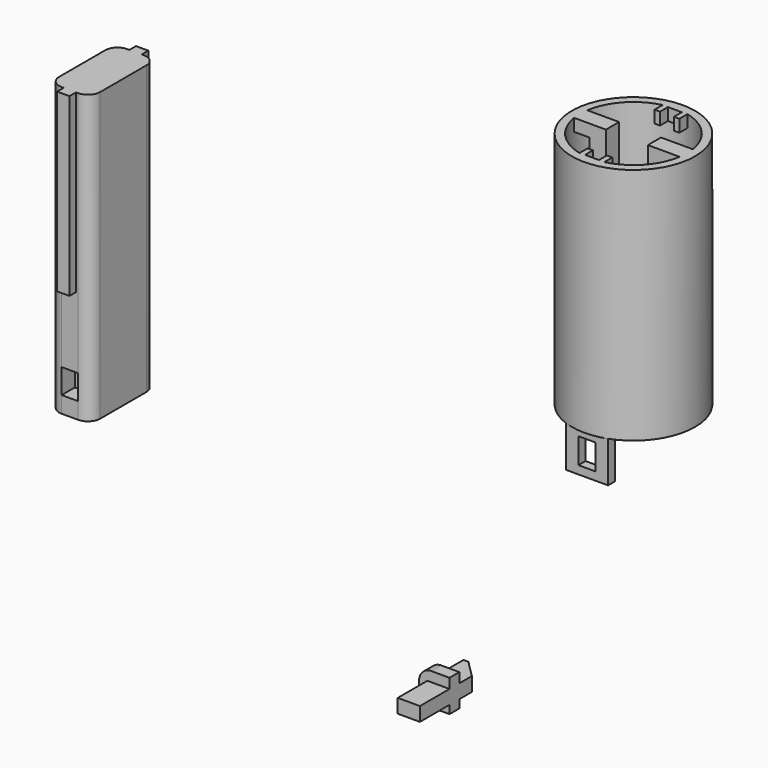
from build123d import *

# Parameters (mm, degrees)
F0_R           = 7.5
F1_DEPTH       = 29
F2_R           = 6.5
F3_DEPTH       = 30
F4_R           = 7.5
F4_R_2         = 6.5
F5_DEPTH       = 2
F7_DEPTH       = 35
F9_DEPTH       = 1.5
F10_W          = 1.5
F10_H          = 1
F11_DEPTH      = 13.6
F13_DEPTH      = 25
F14_R          = 1.5
F15_W          = 1
F15_H          = 3
F16_DEPTH      = 2
F17_W          = 5.1
F17_H          = 1.0742694599
F18_DEPTH      = 5
F19_W          = 2.1
F19_H          = 3.1
F20_DEPTH      = 25
F21_W          = 2.7
F21_H          = 1.7
F22_DEPTH      = 10
F24_DEPTH      = 25
F25_W          = 2
F25_H          = 2
F26_DEPTH      = 25.5
F27_W          = 3.7
F27_H          = 1.5
F28_DEPTH      = 1
F28_DEPTH_BACK = 2.9
F29_R          = 1.5


# Not quite as in the source:
# - a feature names something its author has since deleted; it is built from what else it names


with BuildPart() as f1:
    # F0 (on Top) → F1 (new body)
    with BuildSketch(Plane.XY):
        Circle(F0_R)
    extrude(amount=F1_DEPTH)

    # F2 (on Top) → F3 (cut)
    with BuildSketch(Plane.XY):
        Circle(F2_R)
    extrude(amount=F3_DEPTH, mode=Mode.SUBTRACT)

    # F4 (on face) → F5 (join)
    with BuildSketch(Plane(origin=(0, 0, 0), x_dir=(1, 0, 0), z_dir=(0, 0, -1))):
        Circle(F4_R)
        Circle(F4_R_2, mode=Mode.SUBTRACT)
        Circle(F4_R_2)
    extrude(amount=-F5_DEPTH)

    # F8 (on face) → F9 (join)
    with BuildSketch(Plane.XY.offset(29)):
        with BuildLine():
            Line((-2.55, 1), (-5.9160797831, 1))
            ThreePointArc((-5.9160797831, 1), (-6, 0), (-5.9160797831, -1))
            Line((-5.9160797831, -1), (-2.55, -1))
            Line((-2.55, -1), (-2.55, 1))
        make_face()
        with BuildLine():
            ThreePointArc((5.9160797831, -1), (6, 0), (5.9160797831, 1))
            Line((5.9160797831, 1), (2.55, 1))
            Line((2.55, 1), (2.55, -1))
            Line((2.55, -1), (5.9160797831, -1))
        make_face()
        with BuildLine():
            ThreePointArc((-5.9160797831, -1), (-6, 0), (-5.9160797831, 1))
            Line((-5.9160797831, 1), (-6.4226162893, 1))
            ThreePointArc((-6.4226162893, 1), (-6.4806251967, 0.5014948252), (-6.5, 0))
            ThreePointArc((-6.5, 0), (-6.4806251967, -0.5014948252), (-6.4226162893, -1))
            Line((-6.4226162893, -1), (-5.9160797831, -1))
        make_face()
        with BuildLine():
            ThreePointArc((6.5, 0), (6.4806251967, 0.5014948252), (6.4226162893, 1))
            Line((6.4226162893, 1), (5.9160797831, 1))
            ThreePointArc((5.9160797831, 1), (6, 0), (5.9160797831, -1))
            Line((5.9160797831, -1), (6.4226162893, -1))
            ThreePointArc((6.4226162893, -1), (6.4806251967, -0.5014948252), (6.5, 0))
        make_face()
        with BuildLine():
            ThreePointArc((0, 6.5), (-0.7551127127, 6.4559898382), (-1.5, 6.3245553203))
            Line((-1.5, 6.3245553203), (-1.5, 5.1))
            Line((-1.5, 5.1), (-0.85, 5.1))
            Line((-0.85, 5.1), (-0.85, 6.3))
            Line((-0.85, 6.3), (0.85, 6.3))
            Line((0.85, 6.3), (0.85, 5.1))
            Line((0.85, 5.1), (1.5, 5.1))
            Line((1.5, 5.1), (1.5, 6.3245553203))
            ThreePointArc((1.5, 6.3245553203), (0.7551127127, 6.4559898382), (0, 6.5))
        make_face()
        with BuildLine():
            Line((-1.5, -5.1), (-1.5, -6.3245553203))
            ThreePointArc((-1.5, -6.3245553203), (-0.7551127127, -6.4559898382), (0, -6.5))
            ThreePointArc((0, -6.5), (0.7551127127, -6.4559898382), (1.5, -6.3245553203))
            Line((1.5, -6.3245553203), (1.5, -5.1))
            Line((1.5, -5.1), (0.85, -5.1))
            Line((0.85, -5.1), (0.85, -6.3))
            Line((0.85, -6.3), (-0.85, -6.3))
            Line((-0.85, -6.3), (-0.85, -5.1))
            Line((-0.85, -5.1), (-1.5, -5.1))
        make_face()
    extrude(amount=-F9_DEPTH)

    # F12 (on face) → F13 (cut)
    with BuildSketch(Plane.XY.offset(2)):
        Polygon((-2.55, 5.55), (-2.55, 1), (-2.55, -1), (-2.55, -5.9789213074), (2.55, -5.9789213074), (2.55, -1), (2.55, 1), (2.55, 5.55), (-0.3, 5.55), (-1, 5.55), align=None)
    extrude(amount=-F13_DEPTH, mode=Mode.SUBTRACT)

    # F17 (on face) → F18 (join)
    with BuildSketch(Plane(origin=(0, 0, 0), x_dir=(1, 0, 0), z_dir=(0, 0, -1))):
        with Locations((0, 6.5160560373)):
            Rectangle(F17_W, F17_H)
    extrude(amount=F18_DEPTH)

    # F19 (on face) → F20 (cut)
    with BuildSketch(Plane.XZ.offset(7.0531907673)):
        with Locations((0, -2.45)):
            Rectangle(F19_W, F19_H)
    extrude(amount=-F20_DEPTH, mode=Mode.SUBTRACT)

    # F25 (on face) → F26 (join, through all)
    with BuildSketch(Plane(origin=(0, 0, 27.5), x_dir=(1, 0, 0), z_dir=(0, 0, -1))):
        with Locations((3.55, 0)):
            Rectangle(F25_W, F25_H)
        with Locations((-3.55, 0)):
            Rectangle(F25_W, F25_H)
    extrude(amount=F26_DEPTH)


with BuildPart() as f7:
    # F6 (on Top) → F7 (new body)
    with BuildSketch(Plane.XY):
        Polygon((-42.7104520947, -25.4771374032), (-42.7104520947, -35.4771374032), (-40.9604520947, -35.4771374032), (-40.9604520947, -36.4771374032), (-39.4604520947, -36.4771374032), (-39.4604520947, -35.4771374032), (-37.7104520947, -35.4771374032), (-37.7104520947, -25.4771374032), (-39.4604520947, -25.4771374032), (-39.4604520947, -24.4771374032), (-40.9604520947, -24.4771374032), (-40.9604520947, -25.4771374032), align=None)
    extrude(amount=F7_DEPTH)

    # F10 (on face) → F11 (cut)
    with BuildSketch(Plane(origin=(0, 0, 0), x_dir=(1, 0, 0), z_dir=(0, 0, -1))):
        with Locations((-40.2104520947, 24.9771374032)):
            Rectangle(F10_W, F10_H)
        with Locations((-40.2104520947, 35.9771374032)):
            Rectangle(F10_W, F10_H)
    extrude(amount=-F11_DEPTH, mode=Mode.SUBTRACT)

    # F14
    f14_edges = [f7.edges().sort_by_distance(p)[0] for p in [
        (-42.710452, -25.477137, 17.5),
        (-37.710452, -25.477137, 17.5),
        (-37.710452, -35.477137, 17.5),
        (-42.710452, -35.477137, 17.5),
    ]]
    fillet(f14_edges, radius=F14_R)

    # F15 (on face) → F16 (cut)
    with BuildSketch(Plane.XZ.offset(35.4771374032)):
        with Locations((-40.7104520947, 3.5)):
            Rectangle(F15_W, F15_H)
        with Locations((-39.7104520947, 3.5)):
            Rectangle(F15_W, F15_H)
    extrude(amount=-F16_DEPTH, mode=Mode.SUBTRACT)


with BuildPart() as f22:
    # F21 (on Front) → F22 (new body)
    with BuildSketch(Plane.XZ):
        with Locations((-19.3377515213, -34.9723634064)):
            Rectangle(F21_W, F21_H)
    extrude(amount=F22_DEPTH)

    # F23 (on face) → F24 (cut)
    with BuildSketch(Plane(origin=(0, 0, -35.8223634064), x_dir=(1, 0, 0), z_dir=(0, 0, -1))):
        Polygon((-17.9877515213, 0), (-17.9877515213, 2.1), (-20.0877515213, 0), align=None)
    extrude(amount=-F24_DEPTH, mode=Mode.SUBTRACT)

    # F27 (on face) → F28 (join, two sides)
    with BuildSketch(Plane(origin=(0, 0, -35.8223634064), x_dir=(1, 0, 0), z_dir=(0, 0, -1))) as f28_sk:
        with Locations((-19.8377515213, 4.75)):
            Rectangle(F27_W, F27_H)
    extrude(amount=F28_DEPTH)
    extrude(f28_sk.sketch, amount=-F28_DEPTH_BACK)

    # F29
    f29_edges = [f22.edges().sort_by_distance(p)[0] for p in [
        (-21.687752, -4.75, -36.822363),
        (-21.687752, -4.75, -32.922363),
    ]]
    fillet(f29_edges, radius=F29_R)


solid = Compound([f1.part, f7.part, f22.part])
